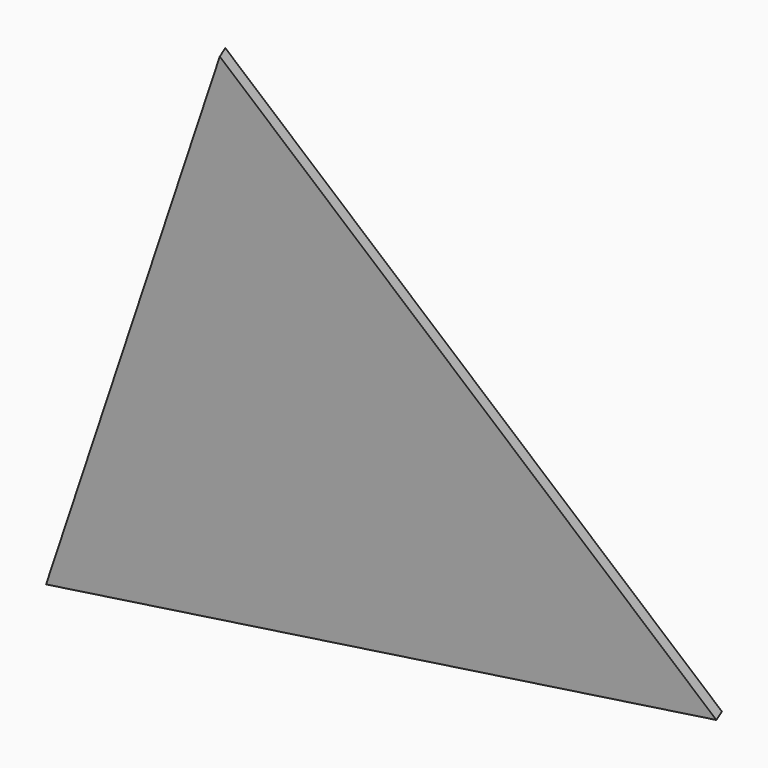
from build123d import *

# Parameters (mm, degrees)
F52_DEPTH = 2.54


# Not quite as in the source:
# - ends of sketch curves that miss each other by under 0.0002 mm in the source are joined


with BuildPart() as f52:
    # F51 (on 3pt) → F52 (new body)
    with BuildSketch(Plane(origin=(-60.6896630699, 226.4969060713, 50.4591961758), x_dir=(0.967459238, 0.2469723498, 0.055020735), z_dir=(0.2530269212, -0.9443093257, -0.2103741298))):
        Polygon((-14.8099569761, 82.2584406081), (-68.5407036056, -47.8326017287), (62.7309768684, -55.2323311128), align=None)
    extrude(amount=-F52_DEPTH)


solid = f52.part
